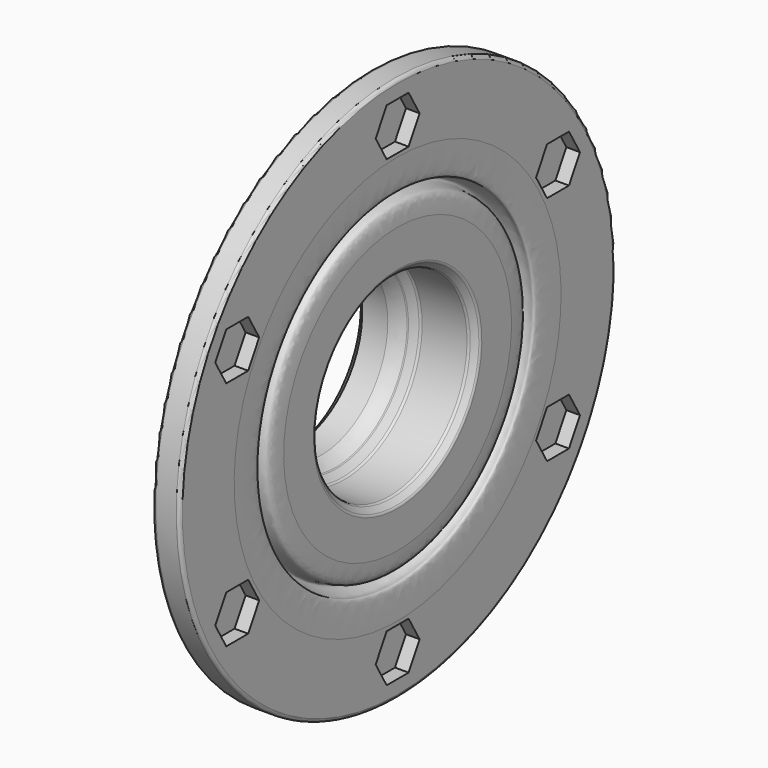
from build123d import *

# Parameters (mm, degrees)
F2_R            = 2
F3_SIZE         = 0.99999
F4_R            = 0.5
F6_R            = 0.5
F9_DEPTH        = 2
F9_COPIES_COUNT = 6
F10_R           = 3


# Not quite as in the source:
# - two fillets or chamfers of one size are made in one step
# - a fillet or chamfer is up to 0.001 mm smaller than in the source, because OpenCascade refuses the exact size
# - a feature of the source that left no trace in its solid (it failed there, or was rolled back) is left out
# - a pattern or mirror of a feature is missing from the dataset's text; its kind, count and spacing are read off the source's solid
# - a feature names something its author has since deleted; it is built from what else it names


with BuildPart() as f1:
    # F0 (on Front) → F1 (revolve)
    with BuildSketch(Plane.XZ):
        with BuildLine():
            Line((-9, 14.25), (0, 14.25))
            Line((0, 14.25), (0, 20.9151750591))
            add(Edge.make_bspline(
                [(0, 20.9151750591), (0, 23.7148292074), (-0.770801608, 23.800552067), (-3.7503474156, 24.206069558), (-0.2333968766, 26.2622078851), (0, 24.1315897015), (0, 30)],
                knots=[0, 0, 0, 0, 0.2726996503, 0.4608875605, 0.6701994511, 1, 1, 1, 1], degree=3))
            Line((0, 30), (0, 40))
            Line((0, 40), (-4, 40))
            Line((-4, 40), (-4, 30))
            Line((-4, 30), (-7.9903741074, 30))
            Line((-7.9903741074, 30), (-10.2543169633, 25.9948689491))
            Line((-10.2543169633, 25.9948689491), (-12.6887708822, 25.9948689491))
            add(Edge.make_bspline(
                [(-12.6887708822, 25.9948689491), (-13.1394076011, 23.8639483866), (-12.8944542608, 22.8394469196), (-8.2436457926, 19), (-12.0932381461, 19)],
                knots=[0, 0, 0, 0, 0.5445750587, 1, 1, 1, 1], degree=3))
            Line((-12.0932381461, 19), (-16, 19))
            Line((-16, 19), (-16, 12.25))
            Line((-16, 12.25), (-9, 12.25))
            Line((-9, 12.25), (-9, 14.25))
        make_face()
    revolve(axis=Axis((-8, 0, 0), (-1, 0, 0)))

    # F2
    f2_edges = [f1.edges().sort_by_distance(p)[0] for p in [
        (-16, 0, -19),
    ]]
    fillet(f2_edges, radius=F2_R)

    # F3 (size 1 in the source; OpenCascade refuses exactly that, so slightly less here)
    f3_edges = [f1.edges().sort_by_distance(p)[0] for p in [
        (-16, 0, -12.25),
        (-9, 0, -12.25),
        (-9, 0, -14.25),
        (0, 0, -14.25),
    ]]
    chamfer(f3_edges, length=F3_SIZE)

    # F4
    f4_edges = [f1.edges().sort_by_distance(p)[0] for p in [
        (-8.00001, 0, -14.25),
    ]]
    fillet(f4_edges, radius=F4_R)

    # F6
    f6_edges = [f1.edges().sort_by_distance(p)[0] for p in [
        (-0.99999, 0, -14.25),
        (0, 0, -15.24999),
        (0, 0, -40),
        (-4, 0, -40),
        (-12.688771, 0, -25.994869),
        (-7.990374, 0, -30),
        (-10.254317, 0, -25.994869),
    ]]
    fillet(f6_edges, radius=F6_R)

    # F8 (on face) → F9 (cut)
    with BuildSketch(Plane.YZ):
        Polygon((-2.0152354679, 37.4818233168), (-4.0304709358, 33.9913330972), (-2.0152354679, 30.5008428776), (2.0152354679, 30.5008428776), (4.0304709358, 33.9913330972), (2.0152354679, 37.4818233168), align=None)
    f9 = extrude(amount=-F9_DEPTH, mode=Mode.SUBTRACT)

    # F9_copies: F9 ×6 about axis
    f9_copies_axis = Axis((0, 0, 0), (1, 0, 0))
    for i in range(1, F9_COPIES_COUNT):
        add(f9.rotate(f9_copies_axis, i * 360 / F9_COPIES_COUNT), mode=Mode.SUBTRACT)

    # F10
    f10_edges = [f1.edges().sort_by_distance(p)[0] for p in [
        (-9.99999, 0, -12.25),
    ]]
    fillet(f10_edges, radius=F10_R)


solid = f1.part
